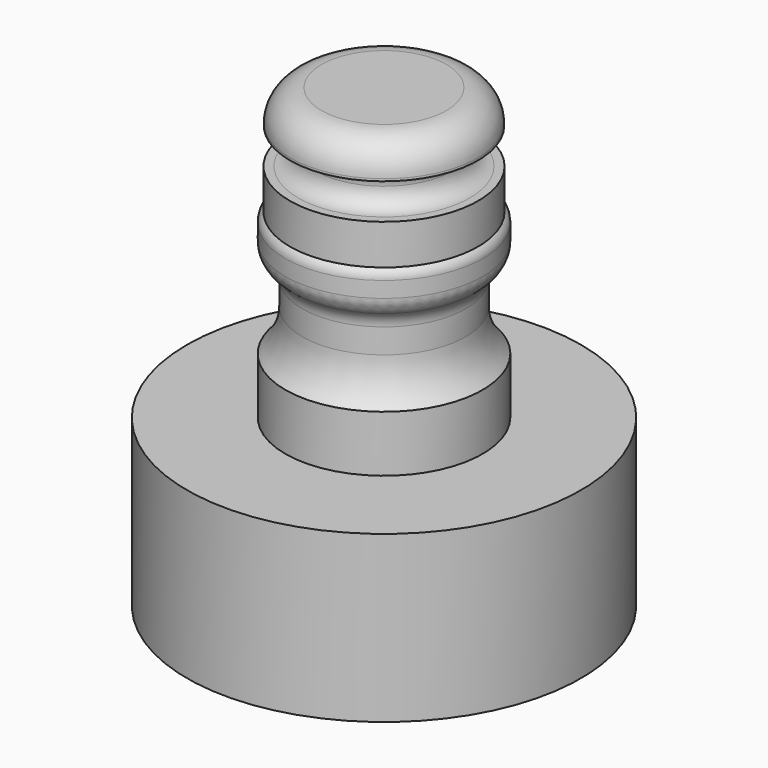
from build123d import *

# Parameters (mm, degrees)
F2_R = 1.49999
F6_R = 1.9156322051
F7_R = 2.6556349186


# Not quite as in the source:
# - a fillet or chamfer that OpenCascade refuses, or shapes differently, is made with other operations: its cross-section is extruded or revolved along the edge and cut away or added
# - a fillet or chamfer is up to 0.001 mm smaller than in the source, because OpenCascade refuses the exact size


with BuildPart() as f1:
    # F0 (on Front) → F1 (revolve)
    with BuildSketch(Plane.XZ):
        Polygon((-16.65, 0), (0, 0), (0, 38.55), (-7.935, 38.55), (-7.935, 35.7), (-5.765, 35.7), (-5.765, 32.7), (-7.96, 32.7), (-7.96, 29.3), (-8.34, 29.3), (-8.34, 26), (-6.92, 26), (-6.92, 18.76), (-8.34, 18.76), (-8.34, 14), (-16.65, 14), align=None)
    revolve(axis=Axis((0, 0, 19.275), (0, 0, -1)))

    # F2 (radius 1.5 in the source; OpenCascade refuses exactly that, so slightly less here)
    f2_edges = [f1.edges().sort_by_distance(p)[0] for p in [
        (5.765, 0, 32.7),
        (5.765, 0, 35.7),
    ]]
    fillet(f2_edges, radius=F2_R)

    # F3: fillet of radius 1.6899494937 on 1 edges, made by hand

    # F3_s1 → F3_t2 (revolve)
    with BuildSketch(Plane.XZ):
        with BuildLine():
            ThreePointArc((-8.34, 26), (-7.3230675447, 25.4271335519), (-6.92, 24.3317504497))
            Line((-6.92, 24.3317504497), (-6.92, 26))
            Line((-6.92, 26), (-8.34, 26))
        make_face()
    revolve(axis=Axis((0, 0, 26), (0, 0, -1)))

    # F4: fillet of radius 0.9656854249 on 1 edges, made by hand

    # F4_s1 → F4_t2 (revolve, cut)
    with BuildSketch(Plane.XZ):
        with BuildLine():
            ThreePointArc((-7.96, 29.3), (-8.2398017842, 28.9605432653), (-8.34, 28.5321973411))
            Line((-8.34, 28.5321973411), (-8.34, 29.3))
            Line((-8.34, 29.3), (-7.96, 29.3))
        make_face()
    revolve(axis=Axis((0, 0, 29.3), (0, 0, -1)), mode=Mode.SUBTRACT)

    # F5: fillet of radius 5 on 1 edges, made by hand

    # F5_s1 → F5_t2 (revolve)
    with BuildSketch(Plane.XZ):
        with BuildLine():
            ThreePointArc((-6.92, 22.2505013966), (-7.2885855292, 20.3663570285), (-8.34, 18.76))
            Line((-8.34, 18.76), (-6.92, 18.76))
            Line((-6.92, 18.76), (-6.92, 22.2505013966))
        make_face()
    revolve(axis=Axis((0, 0, 18.76), (0, 0, -1)))

    # F6
    f6_edges = [f1.edges().sort_by_distance(p)[0] for p in [
        (8.34, 0, 26),
    ]]
    fillet(f6_edges, radius=F6_R)

    # F7
    f7_edges = [f1.edges().sort_by_distance(p)[0] for p in [
        (7.935, 0, 38.55),
    ]]
    fillet(f7_edges, radius=F7_R)


solid = f1.part
